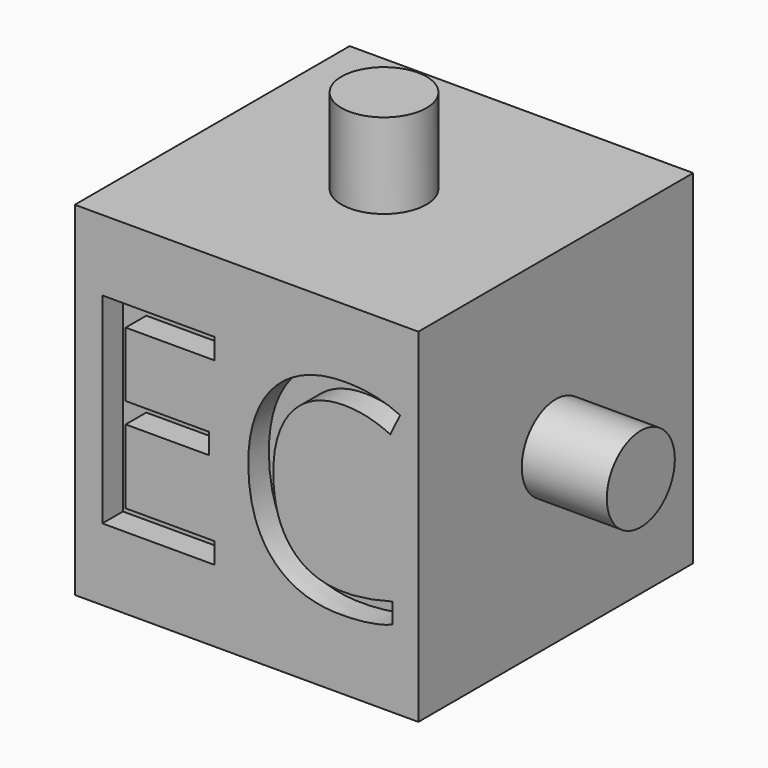
from build123d import *

# Parameters (mm, degrees)
F0_W         = 40
F0_H         = 40
F1_DEPTH     = 40
F2_TEXT_SIZE = 32.7323871628
F3_DEPTH     = 3
F4_R         = 4.95
F5_DEPTH     = 9.9
F6_R         = 4.95
F7_DEPTH     = 9.9
F8_R         = 4.95
F9_DEPTH     = 9.9
F10_R        = 4.95
F11_DEPTH    = 9.9


# Not quite as in the source:
# - Text() gives the source's letters only with a copy of the font that has no kerning and outlines rounded to 1/6400 em; it was checked with that copy


with BuildPart() as f1:
    # F0 (on Front) → F1 (new body)
    with BuildSketch(Plane.XZ):
        with Locations((20, 20)):
            Rectangle(F0_W, F0_H)
    extrude(amount=F1_DEPTH)

    # F2 (on face) → F3 (cut)
    with BuildSketch(Plane.XZ.offset(40)):
        with Locations((0, 8.3828233713)):
            Text('EC', F2_TEXT_SIZE, font='Open Sans', text_align=(TextAlign.LEFT, TextAlign.BOTTOM))
    extrude(amount=-F3_DEPTH, mode=Mode.SUBTRACT)

    # F4 (on face) → F5 (join)
    with BuildSketch(Plane.XY.offset(40)):
        with Locations((20, -20)):
            Circle(F4_R)
    extrude(amount=F5_DEPTH)

    # F6 (on face) → F7 (join)
    with BuildSketch(Plane(origin=(0, 0, 0), x_dir=(0, -1, 0), z_dir=(-1, 0, 0))):
        with Locations((20, 20)):
            Circle(F6_R)
    extrude(amount=F7_DEPTH)

    # F8 (on face) → F9 (join)
    with BuildSketch(Plane.YZ.offset(40)):
        with Locations((-20, 20)):
            Circle(F8_R)
    extrude(amount=F9_DEPTH)

    # F10 (on face) → F11 (join)
    with BuildSketch(Plane(origin=(0, 0, 0), x_dir=(1, 0, 0), z_dir=(0, 0, -1))):
        with Locations((20, 20)):
            Circle(F10_R)
    extrude(amount=F11_DEPTH)


solid = f1.part
